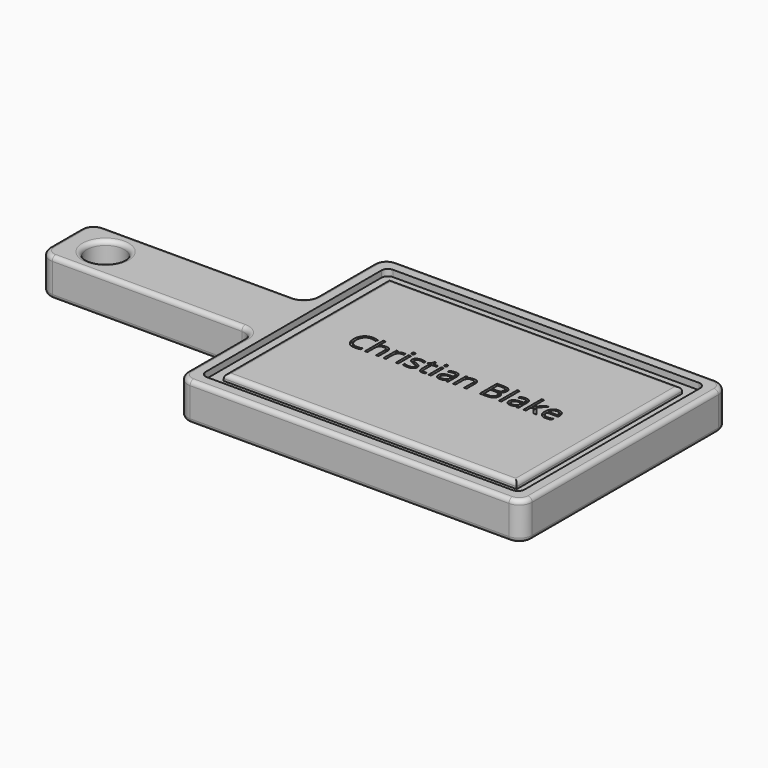
from build123d import *

# Parameters (mm, degrees)
F0_W          = 254
F0_H          = 76.2
F1_DEPTH      = 44.45
F2_R          = 22.225
F4_DEPTH      = 50.8
F7_DEPTH      = 7.62
F8_R          = 7.62
F9_R          = 15.24
F10_R         = 5.08
F11_TEXT_SIZE = 35.6202738153
F12_DEPTH     = 2.54


# Not quite as in the source:
# - Text() gives the source's letters only with a copy of the font that has no kerning and outlines rounded to 1/6400 em; it was checked with that copy


with BuildPart() as f1:
    # F0 (on Top) → F1 (new body)
    with BuildSketch(Plane.XY):
        Polygon((0, 114.3), (0, 0), (406.4, 0), (406.4, 304.8), (0, 304.8), (0, 190.5), align=None)
        with Locations((-127, 152.4)):
            Rectangle(F0_W, F0_H)
    extrude(amount=F1_DEPTH)

    # F2 (on face) → F4 (cut)
    with BuildSketch(Plane.XY.offset(44.45)):
        with Locations((-206.375, 152.4)):
            Circle(F2_R)
    extrude(amount=-F4_DEPTH, mode=Mode.SUBTRACT)

    # F5 (on face) → F7 (cut)
    with BuildSketch(Plane.XY.offset(44.45)):
        Polygon((15.24, 114.3), (15.24, 15.24), (391.16, 15.24), (391.16, 289.56), (15.24, 289.56), (15.24, 190.5), align=None)
        Polygon((30.48, 114.3), (30.48, 190.5), (30.48, 274.32), (375.92, 274.32), (375.92, 30.48), (30.48, 30.48), align=None, mode=Mode.SUBTRACT)
    extrude(amount=-F7_DEPTH, mode=Mode.SUBTRACT)

    # F8
    f8_edges = [f1.edges().sort_by_distance(p)[0] for p in [
        (15.24, 289.56, 40.64),
        (391.16, 289.56, 40.64),
        (15.24, 15.24, 40.64),
        (391.16, 15.24, 40.64),
    ]]
    fillet(f8_edges, radius=F8_R)

    # F9
    f9_edges = [f1.edges().sort_by_distance(p)[0] for p in [
        (0, 0, 22.225),
        (406.4, 0, 22.225),
        (406.4, 304.8, 22.225),
        (0, 304.8, 22.225),
        (0, 190.5, 22.225),
        (-254, 190.5, 22.225),
        (-254, 114.3, 22.225),
        (0, 114.3, 22.225),
    ]]
    fillet(f9_edges, radius=F9_R)

    # F10
    f10_edges = [f1.edges().sort_by_distance(p)[0] for p in [
        (203.2, 304.8, 44.45),
        (203.2, 304.8, 0),
        (203.2, 30.48, 44.45),
        (30.48, 152.4, 44.45),
        (375.92, 152.4, 44.45),
        (203.2, 274.32, 44.45),
        (-228.6, 152.4, 44.45),
        (0, 57.15, 44.45),
        (-4.463693, 109.836307, 44.45),
        (4.463693, 4.463693, 44.45),
        (-127, 114.3, 44.45),
        (203.2, 0, 44.45),
        (-249.536307, 118.763693, 44.45),
        (401.936307, 4.463693, 44.45),
        (-254, 152.4, 44.45),
        (406.4, 152.4, 44.45),
        (-249.536307, 186.036307, 44.45),
        (401.936307, 300.336307, 44.45),
        (-127, 190.5, 44.45),
        (-4.463693, 194.963693, 44.45),
        (4.463693, 300.336307, 44.45),
        (0, 247.65, 44.45),
        (0, 57.15, 0),
        (-4.463693, 109.836307, 0),
        (4.463693, 4.463693, 0),
        (-127, 114.3, 0),
        (203.2, 0, 0),
        (-249.536307, 118.763693, 0),
        (401.936307, 4.463693, 0),
        (-254, 152.4, 0),
        (406.4, 152.4, 0),
        (-249.536307, 186.036307, 0),
        (401.936307, 300.336307, 0),
        (-127, 190.5, 0),
        (-4.463693, 194.963693, 0),
        (4.463693, 300.336307, 0),
        (0, 247.65, 0),
    ]]
    fillet(f10_edges, radius=F10_R)

    # F11 (on face) → F12 (cut)
    with BuildSketch(Plane.XY.offset(44.45)):
        with Locations((78.5275101662, 146.6381251812)):
            Text('Christian Blake', F11_TEXT_SIZE, font='Open Sans', text_align=(TextAlign.LEFT, TextAlign.BOTTOM))
    extrude(amount=-F12_DEPTH, mode=Mode.SUBTRACT)


solid = f1.part
